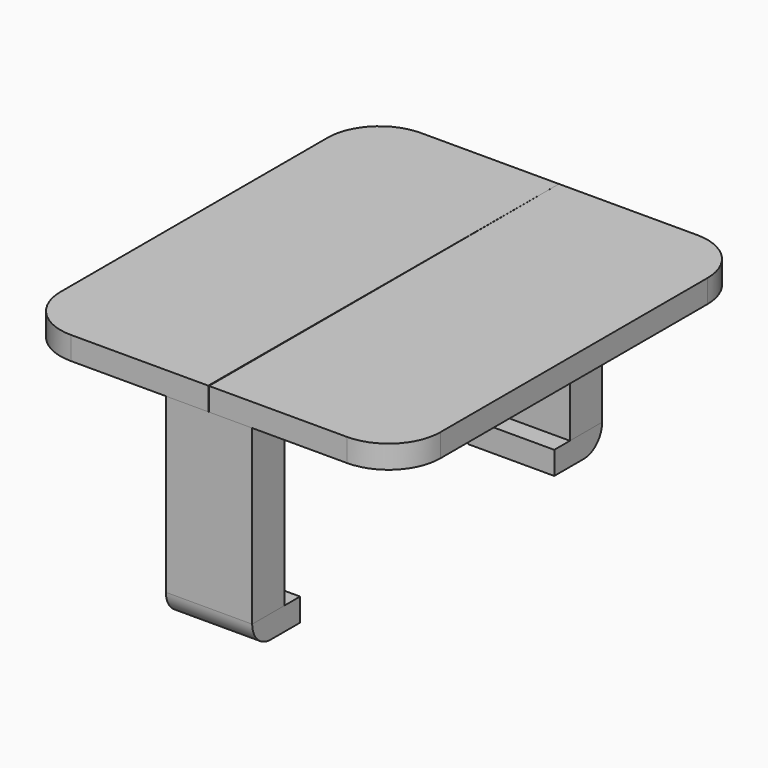
from build123d import *

# Parameters (mm, degrees)
F0_W     = 19.05
F0_H     = 13.208
F1_DEPTH = 5.08
F2_W     = 19.05
F2_H     = 8.89
F3_DEPTH = 38.1
F4_W     = 9.525
F4_H     = 8.89
F5_DEPTH = 5.08
F6_R     = 5.07999
F6_2_R   = 5.07999
F7_R     = 11.43
F7_2_R   = 11.43


# Not quite as in the source:
# - a fillet or chamfer is up to 0.001 mm smaller than in the source, because OpenCascade refuses the exact size


with BuildPart() as f1:
    # F0 (on Top) → F1 (new body)
    with BuildSketch(Plane.XY):
        with Locations((0.1700367264, -10.481657926)):
            Rectangle(F0_W, F0_H)
    extrude(amount=F1_DEPTH)

    # F6#2 (radius 5.08 in the source; OpenCascade refuses exactly that, so slightly less here)
    f6_2_edges = [f1.edges().sort_by_distance(p)[0] for p in [
        (0.170037, -17.085658, 0),
    ]]
    fillet(f6_2_edges, radius=F6_2_R)


with BuildPart() as f1b:
    # F0 (on Top) → F1, piece 2 (new body)
    with BuildSketch(Plane.XY):
        with Locations((0.1700367264, 72.830342074)):
            Rectangle(F0_W, F0_H)
    extrude(amount=F1_DEPTH)

    # F6 (radius 5.08 in the source; OpenCascade refuses exactly that, so slightly less here)
    f6_edges = [f1b.edges().sort_by_distance(p)[0] for p in [
        (0.170037, 79.434342, 0),
    ]]
    fillet(f6_edges, radius=F6_R)


with BuildPart() as f3:
    # F2 (on face) → F3 (new body)
    with BuildSketch(Plane.XY.offset(5.08)):
        with Locations((0.1700367264, -12.640657926)):
            Rectangle(F2_W, F2_H)
    extrude(amount=F3_DEPTH)


with BuildPart() as f3b:
    # F2 (on face) → F3, piece 2 (new body)
    with BuildSketch(Plane.XY.offset(5.08)):
        with Locations((0.1700367264, 74.989342074)):
            Rectangle(F2_W, F2_H)
    extrude(amount=F3_DEPTH)


with BuildPart() as f5:
    # F4 (on face) → F5 (new body)
    with BuildSketch(Plane.XY.offset(43.18)):
        Polygon((9.6950367264, 70.544342074), (0.1700367264, 70.544342074), (0.1700367264, -17.085657926), (42.0800367264, -17.085657926), (42.0800367264, 79.434342074), (9.6950367264, 79.434342074), align=None)
        with Locations((4.9325367264, 74.989342074)):
            Rectangle(F4_W, F4_H)
    extrude(amount=F5_DEPTH)

    # F7
    f7_edges = [f5.edges().sort_by_distance(p)[0] for p in [
        (42.080037, 79.434342, 45.72),
        (42.080037, -17.085658, 45.72),
    ]]
    fillet(f7_edges, radius=F7_R)


with BuildPart() as f5b:
    # F4 (on face) → F5, piece 2 (new body)
    with BuildSketch(Plane.XY.offset(43.18)):
        Polygon((3.6226e-05, -17.085657926), (0.1543787856, 70.544342074), (-9.3549632736, 70.544342074), (-9.3549632736, 79.434342074), (-41.7399632736, 79.434342074), (-41.7399632736, -17.085657926), align=None)
        Polygon((0.1543787856, 70.544342074), (0.1700367264, 79.434342074), (-9.3549632736, 79.434342074), (-9.3549632736, 70.544342074), align=None)
    extrude(amount=F5_DEPTH)

    # F7#2
    f7_2_edges = [f5b.edges().sort_by_distance(p)[0] for p in [
        (-41.739963, 79.434342, 45.72),
        (-41.739963, -17.085658, 45.72),
    ]]
    fillet(f7_2_edges, radius=F7_2_R)


solid = Compound([f1.part, f1b.part, f3.part, f3b.part, f5.part, f5b.part])
